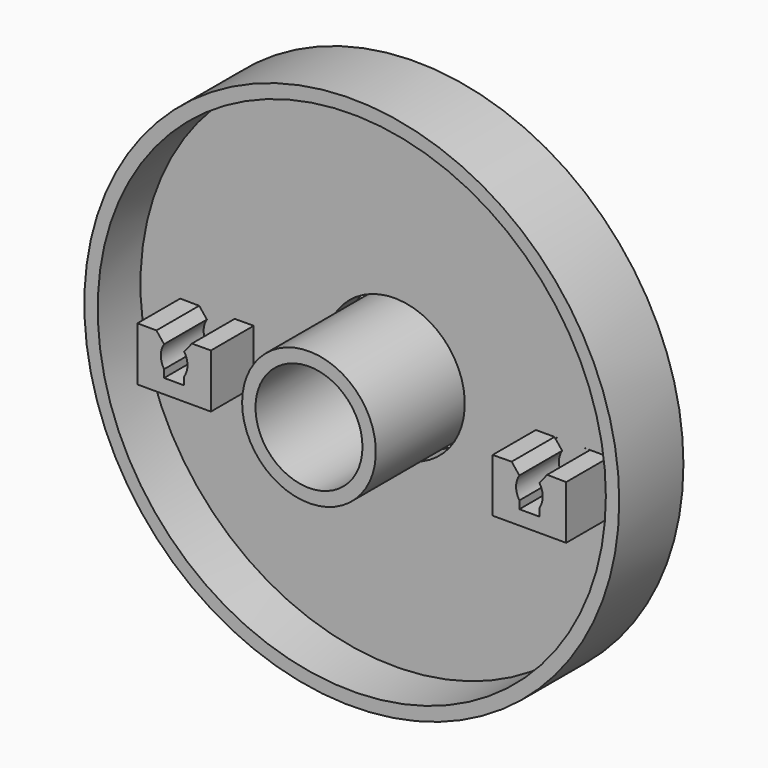
from build123d import *

# Parameters (mm, degrees)
F0_R     = 20
F1_DEPTH = 6
F0_W     = 1.5
F0_H     = 1.0754615068
F2_DEPTH = 2
F3_DEPTH = 10


# Not quite as in the source:
# - a feature names something its author has since deleted; it is built from what else it names


with BuildPart() as f1:
    # F0 (on Front) → F1 (new body)
    with BuildSketch(Plane.XZ):
        Circle(F0_R)
        with BuildLine():
            ThreePointArc((-19, 0), (0, 19), (19, 0))
            ThreePointArc((19, 0), (0, -19), (-19, 0))
        make_face(mode=Mode.SUBTRACT)
    extrude(amount=F1_DEPTH)

    # F0 (on Front) → F2 (join)
    with BuildSketch(Plane.XZ):
        Circle(F0_R)
        with BuildLine():
            ThreePointArc((-19, 0), (0, 19), (19, 0))
            ThreePointArc((19, 0), (0, -19), (-19, 0))
        make_face(mode=Mode.SUBTRACT)
        with BuildLine():
            Line((16.0325318575, 0), (19, 0))
            ThreePointArc((19, 0), (0, 19), (-19, 0))
            Line((-19, 0), (-16.0325318575, 0))
            Line((-16.0325318575, 0), (-14.0325318575, 0))
            Line((-14.0325318575, 0), (-12.5325318575, 0))
            Line((-12.5325318575, 0), (-10.5325318575, 0))
            Line((-10.5325318575, 0), (-7.5, 0))
            ThreePointArc((-7.5, 0), (0, 7.5), (7.5, 0))
            Line((7.5, 0), (10.5325318575, 0))
            Line((10.5325318575, 0), (12.5325318575, 0))
            Line((12.5325318575, 0), (14.0325318575, 0))
            Line((14.0325318575, 0), (16.0325318575, 0))
        make_face()
        with BuildLine():
            ThreePointArc((-19, 0), (0, -19), (19, 0))
            Line((19, 0), (16.0325318575, 0))
            Line((16.0325318575, 0), (16.0325318575, -0.0255133063))
            Line((16.0325318575, -0.0255133063), (16.0325318575, -4.0255133063))
            Line((16.0325318575, -4.0255133063), (14.0325318575, -4.0255133063))
            Line((14.0325318575, -4.0255133063), (12.5325318575, -4.0255133063))
            Line((12.5325318575, -4.0255133063), (10.5325318575, -4.0255133063))
            Line((10.5325318575, -4.0255133063), (10.5325318575, -0.0255133063))
            Line((10.5325318575, -0.0255133063), (10.5325318575, 0))
            Line((10.5325318575, 0), (7.5, 0))
            ThreePointArc((7.5, 0), (0, -7.5), (-7.5, 0))
            Line((-7.5, 0), (-10.5325318575, 0))
            Line((-10.5325318575, 0), (-10.5325318575, -4.0255133063))
            Line((-10.5325318575, -4.0255133063), (-12.5325318575, -4.0255133063))
            Line((-12.5325318575, -4.0255133063), (-14.0325318575, -4.0255133063))
            Line((-14.0325318575, -4.0255133063), (-16.0325318575, -4.0255133063))
            Line((-16.0325318575, -4.0255133063), (-16.0325318575, 0))
            Line((-16.0325318575, 0), (-19, 0))
        make_face()
        with BuildLine():
            Line((-10.5325318575, -4.0255133063), (-10.5325318575, 0))
            Line((-10.5325318575, 0), (-11.9558069244, -0.0073570799))
            Line((-11.9558069244, -0.0073570799), (-12.5325318575, -0.7263235748))
            ThreePointArc((-12.5325318575, -0.7263235748), (-12.2877066772, -1.5473542735), (-12.5325318575, -2.3683849722))
            Line((-12.5325318575, -2.3683849722), (-12.5325318575, -2.9500517994))
            Line((-12.5325318575, -2.9500517994), (-12.5325318575, -4.0255133063))
            Line((-12.5325318575, -4.0255133063), (-10.5325318575, -4.0255133063))
        make_face()
        with BuildLine():
            ThreePointArc((-7.5, 0), (0, -7.5), (7.5, 0))
            Line((7.5, 0), (5.25, 0))
            ThreePointArc((5.25, 0), (0, -5.25), (-5.25, 0))
            Line((-5.25, 0), (-7.5, 0))
        make_face()
        with BuildLine():
            Line((5.25, 0), (7.5, 0))
            ThreePointArc((7.5, 0), (0, 7.5), (-7.5, 0))
            Line((-7.5, 0), (-5.25, 0))
            ThreePointArc((-5.25, 0), (0, 5.25), (5.25, 0))
        make_face()
        with BuildLine():
            Line((-14.0325318575, 0), (-16.0325318575, 0))
            Line((-16.0325318575, 0), (-14.6092567906, -0.0073570799))
            Line((-14.6092567906, -0.0073570799), (-14.0325318575, -0.7263235748))
            ThreePointArc((-14.0325318575, -0.7263235748), (-14.2773570377, -1.5473542735), (-14.0325318575, -2.3683849722))
            Line((-14.0325318575, -2.3683849722), (-14.0325318575, -2.9500517994))
            Line((-14.0325318575, -2.9500517994), (-12.5325318575, -2.9500517994))
            Line((-12.5325318575, -2.9500517994), (-12.5325318575, -2.3683849722))
            ThreePointArc((-12.5325318575, -2.3683849722), (-12.2877066772, -1.5473542735), (-12.5325318575, -0.7263235748))
            Line((-12.5325318575, -0.7263235748), (-11.9558069244, -0.0073570799))
            Line((-11.9558069244, -0.0073570799), (-10.5325318575, 0))
            Line((-10.5325318575, 0), (-12.5325318575, 0))
            Line((-12.5325318575, 0), (-14.0325318575, 0))
        make_face()
        with BuildLine():
            Line((14.6092567906, -0.0073570799), (14.0325318575, 0))
            Line((14.0325318575, 0), (12.5325318575, 0))
            Line((12.5325318575, 0), (11.9558069244, -0.0073570799))
            Line((11.9558069244, -0.0073570799), (12.5325318575, -0.7263235748))
            ThreePointArc((12.5325318575, -0.7263235748), (12.2877066772, -1.5473542735), (12.5325318575, -2.3683849722))
            Line((12.5325318575, -2.3683849722), (12.5325318575, -2.9500517994))
            Line((12.5325318575, -2.9500517994), (14.0325318575, -2.9500517994))
            Line((14.0325318575, -2.9500517994), (14.0325318575, -2.3683849722))
            ThreePointArc((14.0325318575, -2.3683849722), (14.2773570377, -1.5473542735), (14.0325318575, -0.7263235748))
            Line((14.0325318575, -0.7263235748), (14.6092567906, -0.0073570799))
        make_face()
    extrude(amount=F2_DEPTH)


with BuildPart() as f1b:
    # F0 (on Front) → F1, piece 2 (new body)
    with BuildSketch(Plane.XZ):
        with BuildLine():
            Line((-10.5325318575, -4.0255133063), (-10.5325318575, 0))
            Line((-10.5325318575, 0), (-11.9558069244, -0.0073570799))
            Line((-11.9558069244, -0.0073570799), (-12.5325318575, -0.7263235748))
            ThreePointArc((-12.5325318575, -0.7263235748), (-12.2877066772, -1.5473542735), (-12.5325318575, -2.3683849722))
            Line((-12.5325318575, -2.3683849722), (-12.5325318575, -2.9500517994))
            Line((-12.5325318575, -2.9500517994), (-12.5325318575, -4.0255133063))
            Line((-12.5325318575, -4.0255133063), (-10.5325318575, -4.0255133063))
        make_face()
        with Locations((-13.2825318575, -3.4877825528)):
            Rectangle(F0_W, F0_H)
        with BuildLine():
            Line((-14.6092567906, -0.0073570799), (-16.0325318575, 0))
            Line((-16.0325318575, 0), (-16.0325318575, -4.0255133063))
            Line((-16.0325318575, -4.0255133063), (-14.0325318575, -4.0255133063))
            Line((-14.0325318575, -4.0255133063), (-14.0325318575, -2.9500517994))
            Line((-14.0325318575, -2.9500517994), (-14.0325318575, -2.3683849722))
            ThreePointArc((-14.0325318575, -2.3683849722), (-14.2773570377, -1.5473542735), (-14.0325318575, -0.7263235748))
            Line((-14.0325318575, -0.7263235748), (-14.6092567906, -0.0073570799))
        make_face()
    extrude(amount=F1_DEPTH)


with BuildPart() as f1c:
    # F0 (on Front) → F1, piece 3 (new body)
    with BuildSketch(Plane.XZ):
        with BuildLine():
            Line((16.0325318575, -4.0255133063), (16.0325318575, -0.0255133063))
            Line((16.0325318575, -0.0255133063), (14.6092567906, -0.0073570799))
            Line((14.6092567906, -0.0073570799), (14.0325318575, -0.7263235748))
            ThreePointArc((14.0325318575, -0.7263235748), (14.2773570377, -1.5473542735), (14.0325318575, -2.3683849722))
            Line((14.0325318575, -2.3683849722), (14.0325318575, -2.9500517994))
            Line((14.0325318575, -2.9500517994), (14.0325318575, -4.0255133063))
            Line((14.0325318575, -4.0255133063), (16.0325318575, -4.0255133063))
        make_face()
        with BuildLine():
            Line((12.5325318575, -0.7263235748), (11.9558069244, -0.0073570799))
            Line((11.9558069244, -0.0073570799), (10.5325318575, -0.0255133063))
            Line((10.5325318575, -0.0255133063), (10.5325318575, -4.0255133063))
            Line((10.5325318575, -4.0255133063), (12.5325318575, -4.0255133063))
            Line((12.5325318575, -4.0255133063), (12.5325318575, -2.9500517994))
            Line((12.5325318575, -2.9500517994), (12.5325318575, -2.3683849722))
            ThreePointArc((12.5325318575, -2.3683849722), (12.2877066772, -1.5473542735), (12.5325318575, -0.7263235748))
        make_face()
        with Locations((13.2825318575, -3.4877825528)):
            Rectangle(F0_W, F0_H)
    extrude(amount=F1_DEPTH)


with BuildPart() as f3:
    # F0 (on Front) → F3 (new body)
    with BuildSketch(Plane.XZ):
        with BuildLine():
            Line((4, 0), (5, 0))
            ThreePointArc((5, 0), (0, 5), (-5, 0))
            Line((-5, 0), (-4, 0))
            ThreePointArc((-4, 0), (0, 4), (4, 0))
        make_face()
        with BuildLine():
            ThreePointArc((-5, 0), (0, -5), (5, 0))
            Line((5, 0), (4, 0))
            ThreePointArc((4, 0), (0, -4), (-4, 0))
            Line((-4, 0), (-5, 0))
        make_face()
    extrude(amount=F3_DEPTH)


solid = Compound([f1.part, f1b.part, f1c.part, f3.part])
